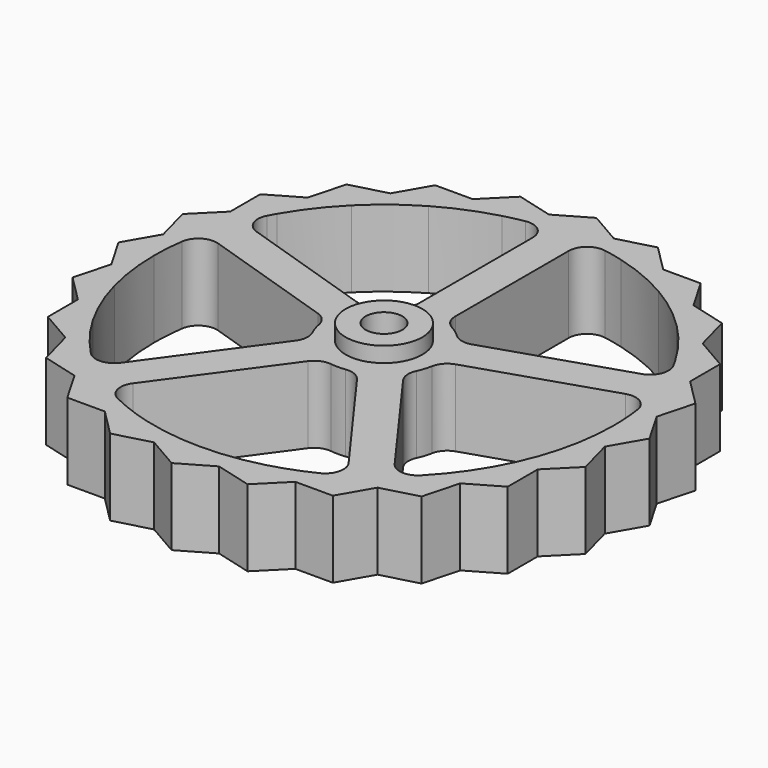
from build123d import *

# Parameters (mm, degrees)
F0_R     = 1
F1_DEPTH = 10
F2_R     = 5
F2_R_2   = 1
F3_DEPTH = 2
F4_R     = 2.4
F5_DEPTH = 3
F6_R     = 5
F7_DEPTH = 8
F8_R     = 2.4


with BuildPart() as f1:
    # F0 (on Top) → F1 (new body)
    with BuildSketch(Plane.XY):
        with BuildLine():
            ThreePointArc((-7.4999226442, -0.0340636396), (-7.1329238722, 2.3176274578), (-6.0475427706, 4.4359019869))
            Line((-6.0475427706, 4.4359019869), (-27.7178340277, 11.4770064395))
            ThreePointArc((-27.7178340277, 11.4770064395), (-28.4085120627, 9.6413921392), (-28.9777747684, 7.7645714286))
            ThreePointArc((-28.9777747684, 7.7645714286), (-29.0764614378, 7.3864328507), (-29.1702139013, 7.0070408129))
            Line((-29.1702139013, 7.0070408129), (-7.4999226442, -0.0340636396))
        make_face()
        with BuildLine():
            Line((-2.35, 0.7635612861), (-2.35, 3.2344975131))
            Line((-2.35, 3.2344975131), (-6.0475427706, 4.4359019869))
            ThreePointArc((-6.0475427706, 4.4359019869), (-7.1329238722, 2.3176274578), (-7.4999226442, -0.0340636396))
            Line((-7.4999226442, -0.0340636396), (-3.8023798736, -1.2354681135))
            Line((-3.8023798736, -1.2354681135), (-2.35, 0.7635612861))
        make_face()
        with BuildLine():
            ThreePointArc((1.9011899368, -1.3812953429), (2.2349828133, -0.7261899368), (2.35, 0))
            ThreePointArc((2.35, 0), (2.2349828133, 0.7261899368), (1.9011899368, 1.3812953429))
            ThreePointArc((1.9011899368, 1.3812953429), (1.3812953429, 1.9011899368), (0.7261899368, 2.2349828133))
            ThreePointArc((0.7261899368, 2.2349828133), (0, 2.35), (-0.7261899368, 2.2349828133))
            ThreePointArc((-0.7261899368, 2.2349828133), (-1.3812953429, 1.9011899368), (-1.9011899368, 1.3812953429))
            ThreePointArc((-1.9011899368, 1.3812953429), (-2.2349828133, 0.7261899368), (-2.35, 0))
            ThreePointArc((-2.35, 0), (-2.2349828133, -0.7261899368), (-1.9011899368, -1.3812953429))
            ThreePointArc((-1.9011899368, -1.3812953429), (-1.3812953429, -1.9011899368), (-0.7261899368, -2.2349828133))
            ThreePointArc((-0.7261899368, -2.2349828133), (0, -2.35), (0.7261899368, -2.2349828133))
            ThreePointArc((0.7261899368, -2.2349828133), (1.3812953429, -1.9011899368), (1.9011899368, -1.3812953429))
        make_face()
        Circle(F0_R, mode=Mode.SUBTRACT)
        with BuildLine():
            Line((-2.35, 3.2344975131), (-2.35, 7.1223240589))
            ThreePointArc((-2.35, 7.1223240589), (-4.4083893922, 6.0676274578), (-6.0475427706, 4.4359019869))
            Line((-6.0475427706, 4.4359019869), (-2.35, 3.2344975131))
        make_face()
        with BuildLine():
            Line((0, 2.470936227), (2.35, 3.2344975131))
            Line((2.35, 3.2344975131), (2.35, 7.1223240589))
            ThreePointArc((2.35, 7.1223240589), (0, 7.5), (-2.35, 7.1223240589))
            Line((-2.35, 7.1223240589), (-2.35, 3.2344975131))
            Line((-2.35, 3.2344975131), (0, 2.470936227))
        make_face()
        with BuildLine():
            ThreePointArc((6.0875869807, -4.3807858602), (7.1329238722, -2.3176274578), (7.4999226442, -0.0340636396))
            Line((7.4999226442, -0.0340636396), (3.8023798736, -1.2354681135))
            Line((3.8023798736, -1.2354681135), (6.0875869807, -4.3807858602))
        make_face()
        with BuildLine():
            Line((-2.2852071071, -7.143376546), (0, -3.9980587993))
            Line((0, -3.9980587993), (-1.4523798736, -1.9990293996))
            Line((-1.4523798736, -1.9990293996), (-3.8023798736, -1.2354681135))
            Line((-3.8023798736, -1.2354681135), (-6.0875869807, -4.3807858602))
            ThreePointArc((-6.0875869807, -4.3807858602), (-4.4083893922, -6.0676274578), (-2.2852071071, -7.143376546))
        make_face()
        with BuildLine():
            ThreePointArc((-7.4999226442, -0.0340636396), (-7.1329238722, -2.3176274578), (-6.0875869807, -4.3807858602))
            Line((-6.0875869807, -4.3807858602), (-3.8023798736, -1.2354681135))
            Line((-3.8023798736, -1.2354681135), (-7.4999226442, -0.0340636396))
        make_face()
        with BuildLine():
            Line((1.9011899368, 1.3812953429), (2.35, 0.7635612861))
            Line((2.35, 0.7635612861), (2.35, 3.2344975131))
            Line((2.35, 3.2344975131), (0, 2.470936227))
            Line((0, 2.470936227), (0.7261899368, 2.2349828133))
            ThreePointArc((0.7261899368, 2.2349828133), (1.3812953429, 1.9011899368), (1.9011899368, 1.3812953429))
        make_face()
        with BuildLine():
            Line((3.8023798736, -1.2354681135), (7.4999226442, -0.0340636396))
            ThreePointArc((7.4999226442, -0.0340636396), (7.499980661, -0.0170318637), (7.5, 0))
            ThreePointArc((7.5, 0), (7.1276423444, 2.3338197467), (6.0475427706, 4.4359019869))
            Line((6.0475427706, 4.4359019869), (2.35, 3.2344975131))
            Line((2.35, 3.2344975131), (2.35, 0.7635612861))
            Line((2.35, 0.7635612861), (3.8023798736, -1.2354681135))
        make_face()
        with BuildLine():
            ThreePointArc((-2.2852071071, -7.143376546), (0, -7.5), (2.2852071071, -7.143376546))
            Line((2.2852071071, -7.143376546), (0, -3.9980587993))
            Line((0, -3.9980587993), (-2.2852071071, -7.143376546))
        make_face()
        with BuildLine():
            Line((-0.7261899368, 2.2349828133), (0, 2.470936227))
            Line((0, 2.470936227), (-2.35, 3.2344975131))
            Line((-2.35, 3.2344975131), (-2.35, 0.7635612861))
            Line((-2.35, 0.7635612861), (-1.9011899368, 1.3812953429))
            ThreePointArc((-1.9011899368, 1.3812953429), (-1.3812953429, 1.9011899368), (-0.7261899368, 2.2349828133))
        make_face()
        with BuildLine():
            Line((1.4523798736, -1.9990293996), (3.8023798736, -1.2354681135))
            Line((3.8023798736, -1.2354681135), (2.35, 0.7635612861))
            Line((2.35, 0.7635612861), (2.35, 0))
            ThreePointArc((2.35, 0), (2.2349828133, -0.7261899368), (1.9011899368, -1.3812953429))
            Line((1.9011899368, -1.3812953429), (1.4523798736, -1.9990293996))
        make_face()
        with BuildLine():
            Line((-3.8023798736, -1.2354681135), (-1.4523798736, -1.9990293996))
            Line((-1.4523798736, -1.9990293996), (-1.9011899368, -1.3812953429))
            ThreePointArc((-1.9011899368, -1.3812953429), (-2.2349828133, -0.7261899368), (-2.35, 0))
            Line((-2.35, 0), (-2.35, 0.7635612861))
            Line((-2.35, 0.7635612861), (-3.8023798736, -1.2354681135))
        make_face()
        with BuildLine():
            Line((6.0875869807, -4.3807858602), (3.8023798736, -1.2354681135))
            Line((3.8023798736, -1.2354681135), (1.4523798736, -1.9990293996))
            Line((1.4523798736, -1.9990293996), (0, -3.9980587993))
            Line((0, -3.9980587993), (2.2852071071, -7.143376546))
            ThreePointArc((2.2852071071, -7.143376546), (4.4083893922, -6.0676274578), (6.0875869807, -4.3807858602))
        make_face()
        with BuildLine():
            Line((2.35, 3.2344975131), (6.0475427706, 4.4359019869))
            ThreePointArc((6.0475427706, 4.4359019869), (4.4083893922, 6.0676274578), (2.35, 7.1223240589))
            Line((2.35, 7.1223240589), (2.35, 3.2344975131))
        make_face()
        with BuildLine():
            Line((0, -3.9980587993), (1.4523798736, -1.9990293996))
            Line((1.4523798736, -1.9990293996), (0.7261899368, -2.2349828133))
            ThreePointArc((0.7261899368, -2.2349828133), (0, -2.35), (-0.7261899368, -2.2349828133))
            Line((-0.7261899368, -2.2349828133), (-1.4523798736, -1.9990293996))
            Line((-1.4523798736, -1.9990293996), (0, -3.9980587993))
        make_face()
        with BuildLine():
            Line((-1.9011899368, -1.3812953429), (-1.4523798736, -1.9990293996))
            Line((-1.4523798736, -1.9990293996), (-0.7261899368, -2.2349828133))
            ThreePointArc((-0.7261899368, -2.2349828133), (-1.3812953429, -1.9011899368), (-1.9011899368, -1.3812953429))
        make_face()
        with BuildLine():
            Line((2.35, 0), (2.35, 0.7635612861))
            Line((2.35, 0.7635612861), (1.9011899368, 1.3812953429))
            ThreePointArc((1.9011899368, 1.3812953429), (2.2349828133, 0.7261899368), (2.35, 0))
        make_face()
        with BuildLine():
            Line((-1.9011899368, 1.3812953429), (-2.35, 0.7635612861))
            Line((-2.35, 0.7635612861), (-2.35, 0))
            ThreePointArc((-2.35, 0), (-2.2349828133, 0.7261899368), (-1.9011899368, 1.3812953429))
        make_face()
        with BuildLine():
            Line((0.7261899368, -2.2349828133), (1.4523798736, -1.9990293996))
            Line((1.4523798736, -1.9990293996), (1.9011899368, -1.3812953429))
            ThreePointArc((1.9011899368, -1.3812953429), (1.3812953429, -1.9011899368), (0.7261899368, -2.2349828133))
        make_face()
        with BuildLine():
            Line((0.7261899368, 2.2349828133), (0, 2.470936227))
            Line((0, 2.470936227), (-0.7261899368, 2.2349828133))
            ThreePointArc((-0.7261899368, 2.2349828133), (0, 2.35), (0.7261899368, 2.2349828133))
        make_face()
        with BuildLine():
            Line((19.4805635237, -22.8146366353), (6.0875869807, -4.3807858602))
            ThreePointArc((6.0875869807, -4.3807858602), (4.4083893922, -6.0676274578), (2.2852071071, -7.143376546))
            Line((2.2852071071, -7.143376546), (15.6781836501, -25.5772273211))
            ThreePointArc((15.6781836501, -25.5772273211), (17.6335575688, -24.2705098312), (19.4805635237, -22.8146366353))
        make_face()
        with BuildLine():
            Line((-15.6781836501, -25.5772273211), (-2.2852071071, -7.143376546))
            ThreePointArc((-2.2852071071, -7.143376546), (-4.4083893922, -6.0676274578), (-6.0875869807, -4.3807858602))
            Line((-6.0875869807, -4.3807858602), (-19.4805635237, -22.8146366353))
            ThreePointArc((-19.4805635237, -22.8146366353), (-17.6335575688, -24.2705098312), (-15.6781836501, -25.5772273211))
        make_face()
        with BuildLine():
            ThreePointArc((-2.35, 7.1223240589), (0, 7.5), (2.35, 7.1223240589))
            Line((2.35, 7.1223240589), (2.35, 29.907816704))
            ThreePointArc((2.35, 29.907816704), (1.1759036909, 29.9769453165), (4.28e-08, 30))
            ThreePointArc((4.28e-08, 30), (-1.1759036481, 29.9769453182), (-2.35, 29.907816704))
            Line((-2.35, 29.907816704), (-2.35, 7.1223240589))
        make_face()
        with BuildLine():
            Line((7.4999226442, -0.0340636396), (29.1702139013, 7.0070408129))
            ThreePointArc((29.1702139013, 7.0070408129), (29.0764614378, 7.3864328507), (28.9777747684, 7.7645714286))
            ThreePointArc((28.9777747684, 7.7645714286), (28.4085120627, 9.6413921392), (27.7178340277, 11.4770064395))
            Line((27.7178340277, 11.4770064395), (6.0475427706, 4.4359019869))
            ThreePointArc((6.0475427706, 4.4359019869), (7.1276423444, 2.3338197467), (7.5, 0))
            ThreePointArc((7.5, 0), (7.499980661, -0.0170318637), (7.4999226442, -0.0340636396))
        make_face()
        with BuildLine():
            ThreePointArc((-14.9999993112, 25.9807625112), (-11.4805025517, 27.716386149), (-7.7645712447, 28.9777748177))
            Line((-7.7645712447, 28.9777748177), (-11.5795677785, 27.9555495773))
            Line((-11.5795677785, 27.9555495773), (-14.9999993112, 25.9807625112))
        make_face()
        Polygon((-15.5291427062, 26.897264165), (-12.4264068712, 30), (-17.3205080757, 30), (-19.7675586779, 25.7615840282), align=None)
        Polygon((-11.5795677785, 27.9555495773), (-8.0384757729, 30), (-12.4264068712, 30), (-15.5291427062, 26.897264165), align=None)
        Polygon((-18.4204322215, 24.0059746497), (-14.9999993112, 25.9807625112), (-11.5795677785, 27.9555495773), (-15.5291427062, 26.897264165), align=None)
        with BuildLine():
            Line((-24.0059746497, 18.4204322215), (-25.9807618629, 15.0000004341))
            ThreePointArc((-25.9807618629, 15.0000004341), (-23.8006000078, 18.2628431321), (-21.2132033232, 21.213203548))
            Line((-21.2132033232, 21.213203548), (-24.0059746497, 18.4204322215))
        make_face()
        Polygon((-26.897264165, 15.5291427062), (-24.0059746497, 18.4204322215), (-21.9615242271, 21.9615242271), (-25.7615840282, 19.7675586779), align=None)
        Polygon((-25.7615840282, 19.7675586779), (-21.9615242271, 21.9615242271), (-19.7675586779, 25.7615840282), (-24.4948974278, 24.4948974278), align=None)
        Polygon((-21.9615242271, 21.9615242271), (-18.4204322215, 24.0059746497), (-15.5291427062, 26.897264165), (-19.7675586779, 25.7615840282), align=None)
        Polygon((-30, 8.0384757729), (-27.9555495773, 11.5795677785), (-26.897264165, 15.5291427062), (-30, 12.4264068712), align=None)
        with BuildLine():
            ThreePointArc((-28.9777747684, 7.7645714286), (-28.4085120627, 9.6413921392), (-27.7178340277, 11.4770064395))
            ThreePointArc((-27.7178340277, 11.4770064395), (-26.9070190067, 13.2669637887), (-25.9807618629, 15.0000004341))
            Line((-25.9807618629, 15.0000004341), (-27.9555495773, 11.5795677785))
            Line((-27.9555495773, 11.5795677785), (-28.9777747684, 7.7645714286))
        make_face()
        Polygon((-30, 12.4264068712), (-26.897264165, 15.5291427062), (-25.7615840282, 19.7675586779), (-30, 17.3205080757), align=None)
        Polygon((-27.9555495773, 11.5795677785), (-25.9807618629, 15.0000004341), (-24.0059746497, 18.4204322215), (-26.897264165, 15.5291427062), align=None)
        with BuildLine():
            ThreePointArc((-21.2132033232, 21.213203548), (-18.2628424917, 23.8006004992), (-14.9999993112, 25.9807625112))
            Line((-14.9999993112, 25.9807625112), (-18.4204322215, 24.0059746497))
            Line((-18.4204322215, 24.0059746497), (-21.2132033232, 21.213203548))
        make_face()
        Polygon((-24.0059746497, 18.4204322215), (-21.2132033232, 21.213203548), (-18.4204322215, 24.0059746497), (-21.9615242271, 21.9615242271), align=None)
        Polygon((-31.0582854123, 0), (-30, 3.9495749276), (-30, 8.0384757729), (-32.1939655491, 4.2384159718), align=None)
        Polygon((-25.7615840282, -19.7675586779), (-26.897264165, -15.5291427062), (-30, -12.4264068712), (-30, -17.3205080757), align=None)
        Polygon((-26.897264165, -15.5291427062), (-27.9555495773, -11.5795677785), (-30, -8.0384757729), (-30, -12.4264068712), align=None)
        Polygon((-30, -12.4264068712), (-30, -8.0384757729), (-32.1939655491, -4.2384159718), (-33.4606521495, -8.9657547217), align=None)
        Polygon((-30, -3.9495749276), (-30, 0), (-30, 3.9495749276), (-31.0582854123, 0), align=None)
        Polygon((-27.9555495773, -11.5795677785), (-28.9777747728, -7.7645714124), (-30, -3.9495749276), (-30, -8.0384757729), align=None)
        Polygon((-32.1939655491, -4.2384159718), (-31.0582854123, 0), (-32.1939655491, 4.2384159718), (-34.6410161514, 0), align=None)
        with BuildLine():
            Line((-27.9555495773, -11.5795677785), (-25.9807625329, -14.9999992737))
            ThreePointArc((-25.9807625329, -14.9999992737), (-27.716386124, -11.4805026119), (-28.9777747728, -7.7645714124))
            Line((-28.9777747728, -7.7645714124), (-27.9555495773, -11.5795677785))
        make_face()
        Polygon((-30, -8.0384757729), (-30, -3.9495749276), (-31.0582854123, 0), (-32.1939655491, -4.2384159718), align=None)
        with BuildLine():
            ThreePointArc((-28.9777747728, -7.7645714124), (-29.7433458372, -3.9157857971), (-30, 0))
            Line((-30, 0), (-30, -3.9495749276))
            Line((-30, -3.9495749276), (-28.9777747728, -7.7645714124))
        make_face()
        Polygon((-32.1939655491, 4.2384159718), (-30, 8.0384757729), (-30, 12.4264068712), (-33.4606521495, 8.9657547217), align=None)
        with BuildLine():
            ThreePointArc((-30, 0), (-29.7918312381, 3.5280010602), (-29.1702139013, 7.0070408129))
            ThreePointArc((-29.1702139013, 7.0070408129), (-29.0764614378, 7.3864328507), (-28.9777747684, 7.7645714286))
            Line((-28.9777747684, 7.7645714286), (-30, 3.9495749276))
            Line((-30, 3.9495749276), (-30, 0))
        make_face()
        Polygon((-30, 3.9495749276), (-28.9777747684, 7.7645714286), (-27.9555495773, 11.5795677785), (-30, 8.0384757729), align=None)
        Polygon((-8.0384757729, -30), (-11.5795677785, -27.9555495773), (-15.5291427062, -26.897264165), (-12.4264068712, -30), align=None)
        with BuildLine():
            ThreePointArc((-14.9999998053, -25.980762226), (-15.3404186754, -25.7812248519), (-15.6781836501, -25.5772273211))
            ThreePointArc((-15.6781836501, -25.5772273211), (-17.6335575688, -24.2705098312), (-19.4805635237, -22.8146366353))
            ThreePointArc((-19.4805635237, -22.8146366353), (-20.3626327899, -22.0309597128), (-21.2132034227, -21.2132034485))
            Line((-21.2132034227, -21.2132034485), (-18.4204322215, -24.0059746497))
            Line((-18.4204322215, -24.0059746497), (-14.9999998053, -25.980762226))
        make_face()
        Polygon((-18.4204322215, -24.0059746497), (-21.2132034227, -21.2132034485), (-24.0059746497, -18.4204322215), (-21.9615242271, -21.9615242271), align=None)
        Polygon((-3.9495749276, -30), (-7.7645716444, -28.9777747106), (-11.5795677785, -27.9555495773), (-8.0384757729, -30), align=None)
        Polygon((-12.4264068712, -30), (-15.5291427062, -26.897264165), (-19.7675586779, -25.7615840282), (-17.3205080757, -30), align=None)
        Polygon((-19.7675586779, -25.7615840282), (-21.9615242271, -21.9615242271), (-25.7615840282, -19.7675586779), (-24.4948974278, -24.4948974278), align=None)
        Polygon((-4.2384159718, -32.1939655491), (-8.0384757729, -30), (-12.4264068712, -30), (-8.9657547217, -33.4606521495), align=None)
        Polygon((-15.5291427062, -26.897264165), (-18.4204322215, -24.0059746497), (-21.9615242271, -21.9615242271), (-19.7675586779, -25.7615840282), align=None)
        Polygon((-11.5795677785, -27.9555495773), (-14.9999998053, -25.980762226), (-18.4204322215, -24.0059746497), (-15.5291427062, -26.897264165), align=None)
        with BuildLine():
            Line((-24.0059746497, -18.4204322215), (-21.2132034227, -21.2132034485))
            ThreePointArc((-21.2132034227, -21.2132034485), (-23.8006004585, -18.2628425448), (-25.9807625329, -14.9999992737))
            Line((-25.9807625329, -14.9999992737), (-24.0059746497, -18.4204322215))
        make_face()
        Polygon((-24.0059746497, -18.4204322215), (-25.9807625329, -14.9999992737), (-27.9555495773, -11.5795677785), (-26.897264165, -15.5291427062), align=None)
        with BuildLine():
            ThreePointArc((-7.7645716444, -28.9777747106), (-11.4805030064, -27.7163859607), (-14.9999998053, -25.980762226))
            Line((-14.9999998053, -25.980762226), (-11.5795677785, -27.9555495773))
            Line((-11.5795677785, -27.9555495773), (-7.7645716444, -28.9777747106))
        make_face()
        Polygon((0, -31.0582854123), (-3.9495749276, -30), (-8.0384757729, -30), (-4.2384159718, -32.1939655491), align=None)
        Polygon((-21.9615242271, -21.9615242271), (-24.0059746497, -18.4204322215), (-26.897264165, -15.5291427062), (-25.7615840282, -19.7675586779), align=None)
        with BuildLine():
            Line((-3.9495749276, -30), (0, -30))
            ThreePointArc((0, -30), (-3.9157859161, -29.7433458215), (-7.7645716444, -28.9777747106))
            Line((-7.7645716444, -28.9777747106), (-3.9495749276, -30))
        make_face()
        Polygon((4.2384159718, -32.1939655491), (0, -31.0582854123), (-4.2384159718, -32.1939655491), (0, -34.6410161514), align=None)
        Polygon((12.4264068712, -30), (15.5291427062, -26.897264165), (11.5795677785, -27.9555495773), (8.0384757729, -30), align=None)
        Polygon((30, -12.4264068712), (26.897264165, -15.5291427062), (25.7615840282, -19.7675586779), (30, -17.3205080757), align=None)
        Polygon((25.7615840282, -19.7675586779), (21.9615242271, -21.9615242271), (19.7675586779, -25.7615840282), (24.4948974278, -24.4948974278), align=None)
        Polygon((19.7675586779, -25.7615840282), (15.5291427062, -26.897264165), (12.4264068712, -30), (17.3205080757, -30), align=None)
        Polygon((8.9657547217, -33.4606521495), (12.4264068712, -30), (8.0384757729, -30), (4.2384159718, -32.1939655491), align=None)
        Polygon((8.0384757729, -30), (3.9495749276, -30), (0, -31.0582854123), (4.2384159718, -32.1939655491), align=None)
        Polygon((21.9615242271, -21.9615242271), (18.4204322215, -24.0059746497), (15.5291427062, -26.897264165), (19.7675586779, -25.7615840282), align=None)
        Polygon((26.897264165, -15.5291427062), (24.0059746497, -18.4204322215), (21.9615242271, -21.9615242271), (25.7615840282, -19.7675586779), align=None)
        Polygon((24.0059746497, -18.4204322215), (21.2132037281, -21.2132031431), (18.4204322215, -24.0059746497), (21.9615242271, -21.9615242271), align=None)
        Polygon((15.5291427062, -26.897264165), (18.4204322215, -24.0059746497), (14.9999995303, -25.9807623847), (11.5795677785, -27.9555495773), align=None)
        Polygon((30, -8.0384757729), (27.9555495773, -11.5795677785), (26.897264165, -15.5291427062), (30, -12.4264068712), align=None)
        Polygon((27.9555495773, -11.5795677785), (25.9807620323, -15.0000001408), (24.0059746497, -18.4204322215), (26.897264165, -15.5291427062), align=None)
        Polygon((11.5795677785, -27.9555495773), (7.7645719804, -28.9777746206), (3.9495749276, -30), (8.0384757729, -30), align=None)
        Polygon((3.9495749276, -30), (0, -30), (-3.9495749276, -30), (0, -31.0582854123), align=None)
        with BuildLine():
            Line((11.5795677785, -27.9555495773), (14.9999995303, -25.9807623847))
            ThreePointArc((14.9999995303, -25.9807623847), (11.4805030204, -27.7163859549), (7.7645719804, -28.9777746206))
            Line((7.7645719804, -28.9777746206), (11.5795677785, -27.9555495773))
        make_face()
        with BuildLine():
            Line((24.0059746497, -18.4204322215), (25.9807620323, -15.0000001408))
            ThreePointArc((25.9807620323, -15.0000001408), (23.8006002852, -18.2628427707), (21.2132037281, -21.2132031431))
            Line((21.2132037281, -21.2132031431), (24.0059746497, -18.4204322215))
        make_face()
        with BuildLine():
            Line((27.9555495773, -11.5795677785), (28.9777749655, -7.7645706931))
            ThreePointArc((28.9777749655, -7.7645706931), (27.716386075, -11.4805027304), (25.9807620323, -15.0000001408))
            Line((25.9807620323, -15.0000001408), (27.9555495773, -11.5795677785))
        make_face()
        with BuildLine():
            Line((3.9495749276, -30), (7.7645719804, -28.9777746206))
            ThreePointArc((7.7645719804, -28.9777746206), (3.9157860885, -29.7433457988), (0, -30))
            Line((0, -30), (3.9495749276, -30))
        make_face()
        with BuildLine():
            Line((18.4204322215, -24.0059746497), (21.2132037281, -21.2132031431))
            ThreePointArc((21.2132037281, -21.2132031431), (20.3626329484, -22.0309595662), (19.4805635237, -22.8146366353))
            ThreePointArc((19.4805635237, -22.8146366353), (17.6335575688, -24.2705098312), (15.6781836501, -25.5772273211))
            ThreePointArc((15.6781836501, -25.5772273211), (15.3404185389, -25.7812249331), (14.9999995303, -25.9807623847))
            Line((14.9999995303, -25.9807623847), (18.4204322215, -24.0059746497))
        make_face()
        Polygon((30, 8.0384757729), (30, 3.9495749276), (31.0582854123, 0), (32.1939655491, 4.2384159718), align=None)
        Polygon((21.9615242271, 21.9615242271), (25.7615840282, 19.7675586779), (24.4948974278, 24.4948974278), (19.7675586779, 25.7615840282), align=None)
        Polygon((30, 12.4264068712), (30, 8.0384757729), (32.1939655491, 4.2384159718), (33.4606521495, 8.9657547217), align=None)
        Polygon((32.1939655491, -4.2384159718), (30, -8.0384757729), (30, -12.4264068712), (33.4606521495, -8.9657547217), align=None)
        Polygon((24.0059746497, 18.4204322215), (26.897264165, 15.5291427062), (25.7615840282, 19.7675586779), (21.9615242271, 21.9615242271), align=None)
        Polygon((26.897264165, 15.5291427062), (30, 12.4264068712), (30, 17.3205080757), (25.7615840282, 19.7675586779), align=None)
        Polygon((31.0582854123, 0), (30, -3.9495749276), (30, -8.0384757729), (32.1939655491, -4.2384159718), align=None)
        Polygon((25.9807618812, 15.0000004024), (27.9555495773, 11.5795677785), (26.897264165, 15.5291427062), (24.0059746497, 18.4204322215), align=None)
        Polygon((27.9555495773, 11.5795677785), (30, 8.0384757729), (30, 12.4264068712), (26.897264165, 15.5291427062), align=None)
        Polygon((30, 3.9495749276), (30, 0), (30, -3.9495749276), (31.0582854123, 0), align=None)
        Polygon((15.5291427062, 26.897264165), (18.4204322215, 24.0059746497), (21.9615242271, 21.9615242271), (19.7675586779, 25.7615840282), align=None)
        Polygon((30, -3.9495749276), (28.9777749655, -7.7645706931), (27.9555495773, -11.5795677785), (30, -8.0384757729), align=None)
        Polygon((32.1939655491, 4.2384159718), (31.0582854123, 0), (32.1939655491, -4.2384159718), (34.6410161514, 0), align=None)
        with BuildLine():
            ThreePointArc((27.7178340277, 11.4770064395), (28.4085120627, 9.6413921392), (28.9777747684, 7.7645714286))
            Line((28.9777747684, 7.7645714286), (27.9555495773, 11.5795677785))
            Line((27.9555495773, 11.5795677785), (25.9807618812, 15.0000004024))
            ThreePointArc((25.9807618812, 15.0000004024), (26.9070190148, 13.2669637724), (27.7178340277, 11.4770064395))
        make_face()
        Polygon((18.4204322215, 24.0059746497), (21.213203064, 21.2132038072), (24.0059746497, 18.4204322215), (21.9615242271, 21.9615242271), align=None)
        Polygon((28.9777747684, 7.7645714286), (30, 3.9495749276), (30, 8.0384757729), (27.9555495773, 11.5795677785), align=None)
        with BuildLine():
            ThreePointArc((15.0000003877, 25.9807618897), (18.2628428394, 23.8006002324), (21.213203064, 21.2132038072))
            Line((21.213203064, 21.2132038072), (18.4204322215, 24.0059746497))
            Line((18.4204322215, 24.0059746497), (15.0000003877, 25.9807618897))
        make_face()
        with BuildLine():
            ThreePointArc((21.213203064, 21.2132038072), (23.8005999073, 18.2628432631), (25.9807618812, 15.0000004024))
            Line((25.9807618812, 15.0000004024), (24.0059746497, 18.4204322215))
            Line((24.0059746497, 18.4204322215), (21.213203064, 21.2132038072))
        make_face()
        with BuildLine():
            Line((30, -3.9495749276), (30, 0))
            ThreePointArc((30, 0), (29.7433458858, -3.9157854279), (28.9777749655, -7.7645706931))
            Line((28.9777749655, -7.7645706931), (30, -3.9495749276))
        make_face()
        with BuildLine():
            ThreePointArc((29.1702139013, 7.0070408129), (29.7918312381, 3.5280010602), (30, 0))
            Line((30, 0), (30, 3.9495749276))
            Line((30, 3.9495749276), (28.9777747684, 7.7645714286))
            ThreePointArc((28.9777747684, 7.7645714286), (29.0764614378, 7.3864328507), (29.1702139013, 7.0070408129))
        make_face()
        Polygon((3.9495749276, 30), (7.7645712665, 28.9777748119), (11.5795677785, 27.9555495773), (8.0384757729, 30), align=None)
        Polygon((-7.7645712447, 28.9777748177), (-3.9495749276, 30), (-8.0384757729, 30), (-11.5795677785, 27.9555495773), align=None)
        with BuildLine():
            ThreePointArc((-2.35, 29.907816704), (-1.1759036481, 29.9769453182), (4.28e-08, 30))
            Line((4.28e-08, 30), (-3.9495749276, 30))
            Line((-3.9495749276, 30), (-7.7645712447, 28.9777748177))
            ThreePointArc((-7.7645712447, 28.9777748177), (-5.078620122, 29.5670021757), (-2.35, 29.907816704))
        make_face()
        Polygon((-12.4264068712, 30), (-8.0384757729, 30), (-4.2384159718, 32.1939655491), (-8.9657547217, 33.4606521495), align=None)
        Polygon((11.5795677785, 27.9555495773), (15.0000003877, 25.9807618897), (18.4204322215, 24.0059746497), (15.5291427062, 26.897264165), align=None)
        Polygon((4.2384159718, 32.1939655491), (8.0384757729, 30), (12.4264068712, 30), (8.9657547217, 33.4606521495), align=None)
        Polygon((12.4264068712, 30), (15.5291427062, 26.897264165), (19.7675586779, 25.7615840282), (17.3205080757, 30), align=None)
        Polygon((8.0384757729, 30), (11.5795677785, 27.9555495773), (15.5291427062, 26.897264165), (12.4264068712, 30), align=None)
        Polygon((-4.2384159718, 32.1939655491), (0, 31.0582854123), (4.2384159718, 32.1939655491), (0, 34.6410161514), align=None)
        Polygon((0, 31.0582854123), (3.9495749276, 30), (8.0384757729, 30), (4.2384159718, 32.1939655491), align=None)
        Polygon((-8.0384757729, 30), (-3.9495749276, 30), (0, 31.0582854123), (-4.2384159718, 32.1939655491), align=None)
        with BuildLine():
            ThreePointArc((7.7645712665, 28.9777748119), (11.4805031363, 27.7163859068), (15.0000003877, 25.9807618897))
            Line((15.0000003877, 25.9807618897), (11.5795677785, 27.9555495773))
            Line((11.5795677785, 27.9555495773), (7.7645712665, 28.9777748119))
        make_face()
        Polygon((-3.9495749276, 30), (4.28e-08, 30), (3.9495749276, 30), (0, 31.0582854123), align=None)
        with BuildLine():
            ThreePointArc((4.28e-08, 30), (1.1759036909, 29.9769453165), (2.35, 29.907816704))
            ThreePointArc((2.35, 29.907816704), (5.0786201331, 29.5670021738), (7.7645712665, 28.9777748119))
            Line((7.7645712665, 28.9777748119), (3.9495749276, 30))
            Line((3.9495749276, 30), (4.28e-08, 30))
        make_face()
    extrude(amount=F1_DEPTH)

    # F2 (on face) → F3 (join)
    with BuildSketch(Plane.XY.offset(10)):
        Circle(F2_R)
        Circle(F2_R_2, mode=Mode.SUBTRACT)
    extrude(amount=F3_DEPTH)

    # F4 (on face) → F5 (cut)
    with BuildSketch(Plane.XY.offset(12)):
        Circle(F4_R)
    extrude(amount=-F5_DEPTH, mode=Mode.SUBTRACT)

    # F6 (on face) → F7 (cut)
    with BuildSketch(Plane(origin=(0, 0, 0), x_dir=(1, 0, 0), z_dir=(0, 0, -1))):
        Circle(F6_R)
    extrude(amount=-F7_DEPTH, mode=Mode.SUBTRACT)

    # F8
    f8_edges = [f1.edges().sort_by_distance(p)[0] for p in [
        (29.170214, 7.007041, 5),
        (7.499923, -0.034064, 5),
        (6.087587, -4.380786, 5),
        (19.480564, -22.814637, 5),
        (15.678184, -25.577227, 5),
        (-6.087587, -4.380786, 5),
        (-2.285207, -7.143377, 5),
        (2.285207, -7.143377, 5),
        (-15.678184, -25.577227, 5),
        (-19.480564, -22.814637, 5),
        (-29.170214, 7.007041, 5),
        (-27.717834, 11.477006, 5),
        (-2.35, 29.907817, 5),
        (2.35, 29.907817, 5),
        (27.717834, 11.477006, 5),
        (6.047543, 4.435902, 5),
        (2.35, 7.122324, 5),
        (-2.35, 7.122324, 5),
        (-6.047543, 4.435902, 5),
        (-7.499923, -0.034064, 5),
    ]]
    fillet(f8_edges, radius=F8_R)


solid = f1.part
